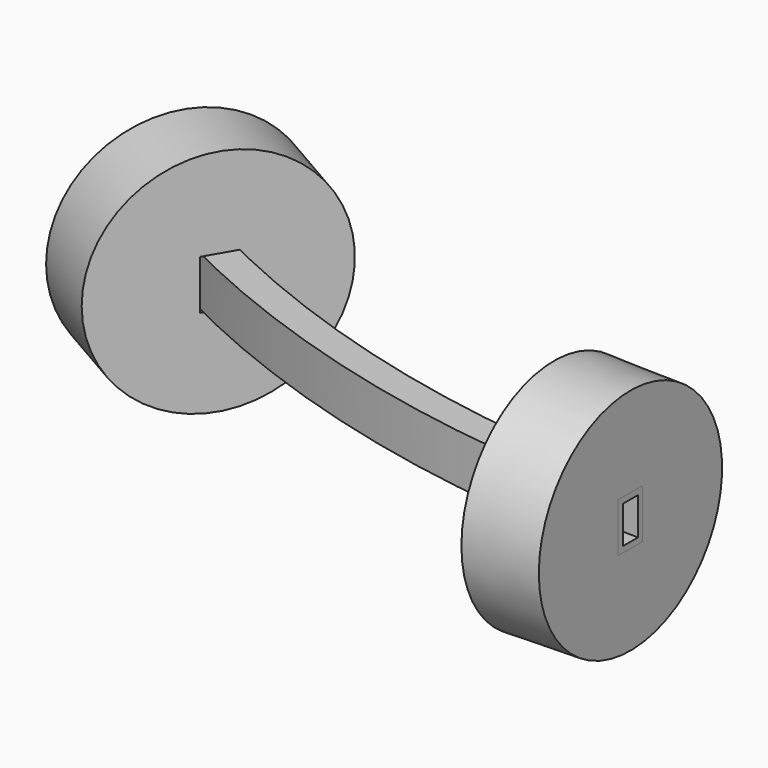
from build123d import *

# Parameters (mm, degrees)
F4_W     = 2.55
F4_H     = 4.1
F4_W_2   = 1.55
F4_H_2   = 3.1
F3_W     = 2.55
F3_H     = 4.1
F3_W_2   = 1.55
F3_H_2   = 3.1
F3_R     = 9.525
F7_DEPTH = 6.35
F4_R     = 9.525
F8_DEPTH = 6.35
F8_TAPER = -1


# Not quite as in the source:
# - a feature of the source that left no trace in its solid (it failed there, or was rolled back) is left out


with BuildPart() as f5:
    # F5: sweep along a path in F0
    with BuildLine(Plane.XY) as f5_path:
        ThreePointArc((-21.9970452561, 12.7), (0.8654840123, 3.2300303069), (25.4, 0))
    # F4 (on line) + F3 (on line) → F5 (sweep)
    with BuildSketch(Plane(origin=(25.4, 0, 0), x_dir=(0, -1, 0), z_dir=(-1, 0, 0))):
        Rectangle(F4_W, F4_H)
        Rectangle(F4_W_2, F4_H_2, mode=Mode.SUBTRACT)
    with BuildSketch(Plane(origin=(-21.9970452561, 12.7, 0), x_dir=(-0.5, -0.8660254038, 0), z_dir=(-0.8660254038, 0.5, 0))):
        Rectangle(F3_W, F3_H)
        Rectangle(F3_W_2, F3_H_2, mode=Mode.SUBTRACT)
    sweep(path=f5_path.line)

    # F4 (on line) → F8 (join)
    with BuildSketch(Plane(origin=(25.4, 0, 0), x_dir=(0, -1, 0), z_dir=(-1, 0, 0))):
        Circle(F4_R)
        Rectangle(F4_W, F4_H, mode=Mode.SUBTRACT)
    extrude(amount=F8_DEPTH, taper=F8_TAPER)


with BuildPart() as f7:
    # F3 (on line) → F7 (new body)
    with BuildSketch(Plane(origin=(-21.9970452561, 12.7, 0), x_dir=(-0.5, -0.8660254038, 0), z_dir=(-0.8660254038, 0.5, 0))):
        Circle(F3_R)
        Rectangle(F3_W, F3_H, mode=Mode.SUBTRACT)
    extrude(amount=-F7_DEPTH)


solid = Compound([f5.part, f7.part])
